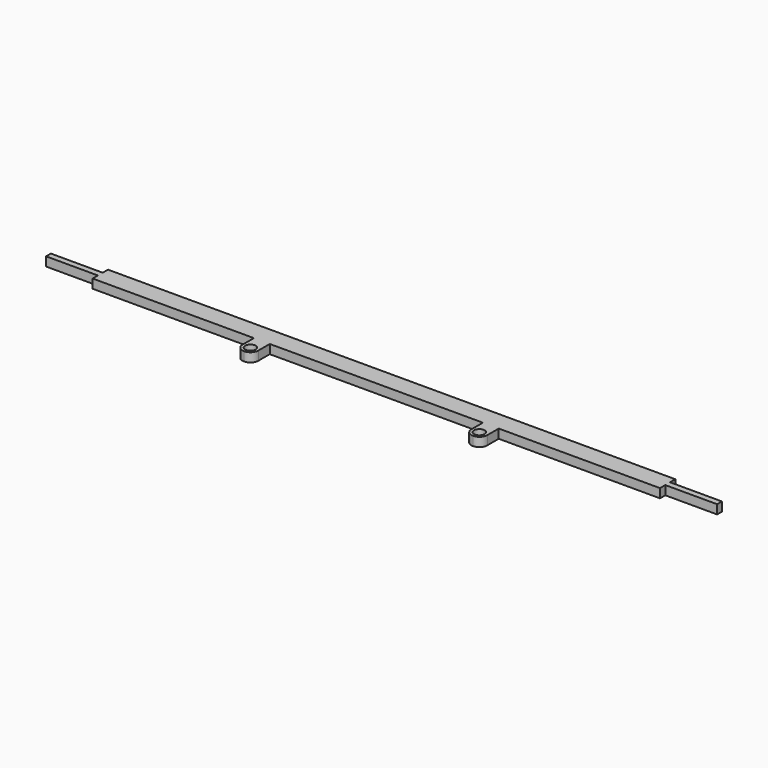
from build123d import *

# Parameters (mm, degrees)
F0_W     = 259.72
F0_H     = 6.4
F1_DEPTH = 3
F3_DEPTH = 3
F4_R     = 2.63999
F5_R     = 1.75
F5_W     = 17.25
F5_H     = 2.2
F6_DEPTH = 3.001
F7_W     = 31.12
F7_H     = 2
F8_DEPTH = 3.001


# Not quite as in the source:
# - a fillet or chamfer is up to 0.001 mm smaller than in the source, because OpenCascade refuses the exact size
# - ends of sketch curves that miss each other by under 0.0002 mm in the source are joined


with BuildPart() as f1:
    # F0 (on Top) → F1 (new body)
    with BuildSketch(Plane.XY):
        Rectangle(F0_W, F0_H)
    extrude(amount=F1_DEPTH)

    # F2 (on Top) → F3 (join)
    with BuildSketch(Plane.XY):
        with BuildLine():
            Line((129.86, -10.59), (129.86, -3.2))
            Line((129.86, -3.2), (124.58, -3.2))
            Line((124.58, -3.2), (124.58, -7.95))
            Line((124.58, -7.95), (125.47, -7.95))
            ThreePointArc((125.47, -7.95), (127.22, -6.2), (128.97, -7.95))
            ThreePointArc((128.97, -7.95), (128.4574368671, -9.1874368671), (127.22, -9.7))
            Line((127.22, -9.7), (127.22, -10.59))
            Line((127.22, -10.59), (129.86, -10.59))
        make_face()
        with BuildLine():
            Line((125.47, -7.95), (124.58, -7.95))
            Line((124.58, -7.95), (124.58, -10.59))
            Line((124.58, -10.59), (127.22, -10.59))
            Line((127.22, -10.59), (127.22, -9.7))
            ThreePointArc((127.22, -9.7), (125.9825631329, -9.1874368671), (125.47, -7.95))
        make_face()
        Polygon((53.66, -10.59), (53.66, -3.2), (48.38, -3.2), (48.38, -7.95), (48.38, -10.59), align=None)
        with BuildLine():
            ThreePointArc((52.77, -7.95), (51.02, -9.7), (49.27, -7.95))
            ThreePointArc((49.27, -7.95), (51.02, -6.2), (52.77, -7.95))
        make_face(mode=Mode.SUBTRACT)
        Polygon((-22.54, -3.2), (-27.82, -3.2), (-27.82, -7.95), (-27.82, -10.59), (-22.54, -10.59), align=None)
        with BuildLine():
            ThreePointArc((-23.43, -7.95), (-25.18, -9.7), (-26.93, -7.95))
            ThreePointArc((-26.93, -7.95), (-25.18, -6.2), (-23.43, -7.95))
        make_face(mode=Mode.SUBTRACT)
    extrude(amount=F3_DEPTH)

    # F4 (radius 2.64 in the source; OpenCascade refuses exactly that, so slightly less here)
    f4_edges = [f1.edges().sort_by_distance(p)[0] for p in [
        (48.38, -10.59, 1.5),
        (53.66, -10.59, 1.5),
        (124.58, -10.59, 1.5),
        (129.86, -10.59, 1.5),
        (-27.82, -10.59, 1.5),
        (-22.54, -10.59, 1.5),
    ]]
    fillet(f4_edges, radius=F4_R)

    # F5 (on face) → F6 (cut, through all)
    with BuildSketch(Plane.XY.offset(3)):
        with BuildLine():
            Line((124.58, 3.2), (124.58, 1))
            Line((124.58, 1), (124.58, -1))
            Line((124.58, -1), (124.58, -3.2))
            Line((124.58, -3.2), (124.58, -7.95001))
            ThreePointArc((124.58, -7.95001), (125.3532351687, -9.8167648313), (127.21999, -10.59))
            ThreePointArc((127.21999, -10.59), (129.0867648313, -9.8167648313), (129.86, -7.95001))
            Line((129.86, -7.95001), (129.86, 3.2))
            Line((129.86, 3.2), (124.58, 3.2))
        make_face()
        with Locations((127.22, -7.95)):
            Circle(F5_R, mode=Mode.SUBTRACT)
        with Locations((115.955, 2.1)):
            Rectangle(F5_W, F5_H)
        with Locations((115.955, -2.1)):
            Rectangle(F5_W, F5_H)
    extrude(amount=-F6_DEPTH, mode=Mode.SUBTRACT)

    # F7 (on face) → F8 (cut, through all)
    with BuildSketch(Plane.XY.offset(3)):
        Polygon((-129.86, 3.2), (-129.86, 1), (-98.74, 1), (-81.49, 1), (-81.49, 3.2), align=None)
        Polygon((-129.86, -1), (-129.86, -3.2), (-81.49, -3.2), (-81.49, -1), (-98.74, -1), align=None)
        with Locations((-114.3, 0)):
            Rectangle(F7_W, F7_H)
    extrude(amount=-F8_DEPTH, mode=Mode.SUBTRACT)


solid = f1.part
